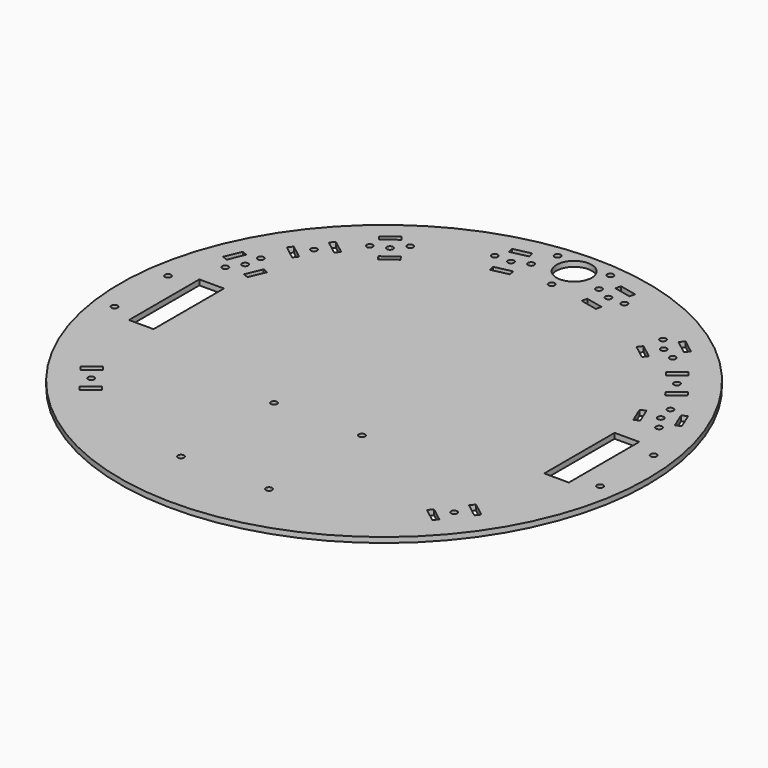
from build123d import *

# Parameters (mm, degrees)
F0_R     = 150
F0_R_2   = 1.75
F0_W     = 14
F0_H     = 50
F1_DEPTH = 3
F2_R     = 1.75
F3_DEPTH = 3
F4_R     = 1.75
F4_R_2   = 10
F5_DEPTH = 3
F6_R     = 1.75
F7_DEPTH = 25
F9_D     = 3.5


# Not quite as in the source:
# - a feature names something its author has since deleted; it is built from what else it names


with BuildPart() as f1:
    # F0 (on Top) → F1 (new body)
    with BuildSketch(Plane.XY):
        Circle(F0_R)
        with Locations((-138, -19)):
            Circle(F0_R_2, mode=Mode.SUBTRACT)
        with Locations((138, -19)):
            Circle(F0_R_2, mode=Mode.SUBTRACT)
        with Locations((-118, 0)):
            Rectangle(F0_W, F0_H, mode=Mode.SUBTRACT)
        with Locations((-138, 19)):
            Circle(F0_R_2, mode=Mode.SUBTRACT)
        with Locations((118, 0)):
            Rectangle(F0_W, F0_H, mode=Mode.SUBTRACT)
        with Locations((138, 19)):
            Circle(F0_R_2, mode=Mode.SUBTRACT)
    extrude(amount=F1_DEPTH)

    # F2 (on face) → F3 (cut, through all)
    with BuildSketch(Plane.XY.offset(3)):
        with Locations((-123.2603204027, 41.3145666106)):
            Circle(F2_R)
        with Locations((-116.3720186201, 57.9443981958)):
            Circle(F2_R)
        with Locations((-86.089285442, 97.4096244325)):
            Circle(F2_R)
        with Locations((-71.8089253168, 108.3673301546)):
            Circle(F2_R)
        with Locations((-36.8563036221, 124.6660053235)):
            Circle(F2_R)
        with Locations((-19.2829754939, 128.5619183744)):
            Circle(F2_R)
        with Locations((19.2829754939, 128.5619183744)):
            Circle(F2_R)
        with Locations((36.8563036221, 124.6660053235)):
            Circle(F2_R)
        with Locations((71.8089253168, 108.3673301546)):
            Circle(F2_R)
        with Locations((86.089285442, 97.4096244325)):
            Circle(F2_R)
        with Locations((116.3720186201, 57.9443981958)):
            Circle(F2_R)
        with Locations((123.2603204027, 41.3145666106)):
            Circle(F2_R)
        Polygon((-126.5058378572, 57.8123947613), (-130.3326721809, 48.5735994362), (-127.3762576769, 47.3490124526), (-123.5494233532, 56.5878077777), align=None)
        Polygon((-105.810936329, 49.2402858763), (-108.767350833, 50.4648728599), (-112.5941851567, 41.2260775348), (-109.6377706526, 40.0014905512), align=None)
        with Locations((-118.0718042549, 48.9069426563)):
            Circle(F2_R)
        Polygon((-86.6365687608, 104.6935764665), (-78.7030353579, 110.7811907566), (-80.6510719308, 113.3199214455), (-88.5846053337, 107.2323071554), align=None)
        with Locations((-77.7997106273, 101.3905568892)):
            Circle(F2_R)
        Polygon((-67.014815921, 95.548806623), (-68.9628524938, 98.0875373119), (-76.8963858967, 91.9999230218), (-74.9483493239, 89.4611923329), align=None)
        Polygon((80.6510719308, 113.3199214455), (78.7030353579, 110.7811907566), (86.6365687608, 104.6935764665), (88.5846053337, 107.2323071554), align=None)
        with Locations((77.7997106273, 101.3905568892)):
            Circle(F2_R)
        Polygon((67.014815921, 95.548806623), (74.9483493239, 89.4611923329), (76.8963858967, 91.9999230218), (68.9628524938, 98.0875373119), align=None)
        Polygon((123.5494233532, 56.5878077777), (127.3762576769, 47.3490124526), (130.3326721809, 48.5735994362), (126.5058378572, 57.8123947613), align=None)
        with Locations((118.0718042549, 48.9069426563)):
            Circle(F2_R)
        Polygon((105.810936329, 49.2402858763), (109.6377706526, 40.0014905512), (112.5941851567, 41.2260775348), (108.767350833, 50.4648728599), align=None)
        Polygon((-25.2036263018, 136.7873430594), (-34.966586373, 134.62294692), (-34.2739796084, 131.4987996972), (-24.5110195372, 133.6631958366), align=None)
        with Locations((-27.6609826613, 124.7706297099)):
            Circle(F2_R)
        Polygon((-21.0479857142, 118.0424597227), (-30.8109457854, 115.8780635833), (-30.1183390208, 112.7539163605), (-20.3553789496, 114.9183124999), align=None)
        Polygon((34.966586373, 134.62294692), (25.2036263018, 136.7873430594), (24.5110195372, 133.6631958366), (34.2739796084, 131.4987996972), align=None)
        with Locations((27.6609826613, 124.7706297099)):
            Circle(F2_R)
        Polygon((30.1183390208, 112.7539163605), (30.8109457854, 115.8780635833), (21.0479857142, 118.0424597227), (20.3553789496, 114.9183124999), align=None)
    extrude(amount=-F3_DEPTH, mode=Mode.SUBTRACT)

    # F4 (on face) → F5 (cut, through all)
    with BuildSketch(Plane.XY.offset(3)):
        with Locations((-15, 142)):
            Circle(F4_R)
        with Locations((15, 142)):
            Circle(F4_R)
        with Locations((0, 119)):
            Circle(F4_R)
        with Locations((0, 135)):
            Circle(F4_R_2)
    extrude(amount=-F5_DEPTH, mode=Mode.SUBTRACT)

    # F6 (on face) → F7 (cut)
    with BuildSketch(Plane.XY.offset(3)):
        Polygon((-105.9872955413, -67.2096212148), (-113.9208289442, -73.2972355049), (-111.9727923714, -75.8359661938), (-104.0392589685, -69.7483519038), align=None)
        with Locations((-103.1359342379, -79.1389857711)):
            Circle(F6_R)
        Polygon((-92.3510395315, -84.9807360374), (-94.2990761043, -82.4420053484), (-102.2326095072, -88.5296196385), (-100.2845729344, -91.0683503274), align=None)
        Polygon((92.3510395315, -84.9807360374), (100.2845729344, -91.0683503274), (102.2326095072, -88.5296196385), (94.2990761043, -82.4420053484), align=None)
        with Locations((103.1359342379, -79.1389857711)):
            Circle(F6_R)
        Polygon((105.9872955413, -67.2096212148), (104.0392589685, -69.7483519038), (111.9727923714, -75.8359661938), (113.9208289442, -73.2972355049), align=None)
        Polygon((111.9727923714, 75.8359661938), (104.0392589685, 69.7483519038), (105.9872955413, 67.2096212148), (113.9208289442, 73.2972355049), align=None)
        with Locations((103.1359342379, 79.1389857711)):
            Circle(F6_R)
        Polygon((94.2990761043, 82.4420053484), (102.2326095072, 88.5296196385), (100.2845729344, 91.0683503274), (92.3510395315, 84.9807360374), align=None)
        Polygon((-92.3510395315, 84.9807360374), (-100.2845729344, 91.0683503274), (-102.2326095072, 88.5296196385), (-94.2990761043, 82.4420053484), align=None)
        with Locations((-103.1359342379, 79.1389857711)):
            Circle(F6_R)
        Polygon((-111.9727923714, 75.8359661938), (-113.9208289442, 73.2972355049), (-105.9872955413, 67.2096212148), (-104.0392589685, 69.7483519038), align=None)
    extrude(amount=-F7_DEPTH, mode=Mode.SUBTRACT)

    # F9 (through all)
    with Locations(Plane.XY.offset(3)):
        with Locations((-25, -47), (25, -47), (25, -113), (-25, -113)):
            Hole(F9_D / 2)


solid = f1.part
